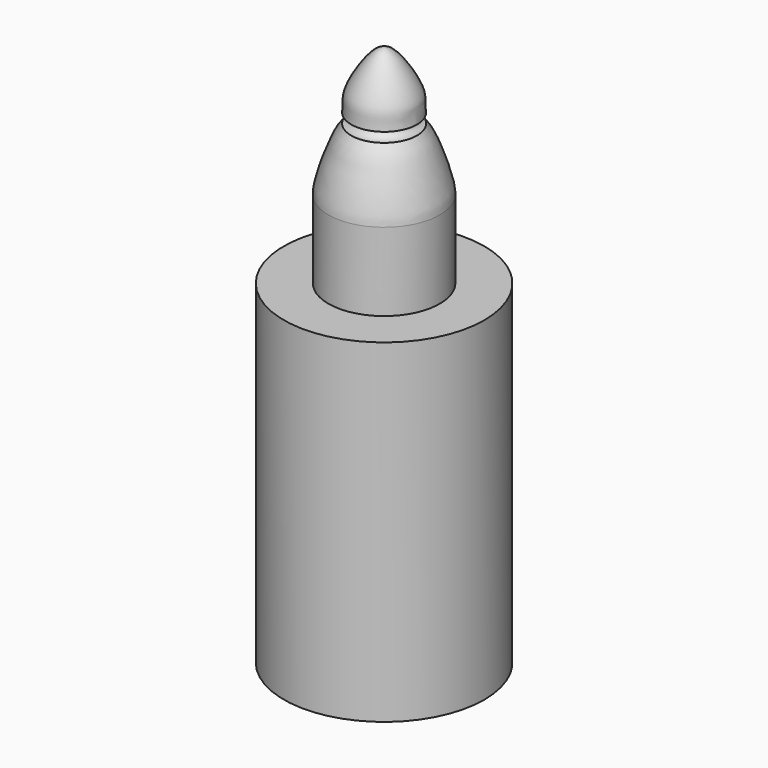
from build123d import *

# Parameters (mm, degrees)
F0_R     = 4.5
F1_DEPTH = 15


# Not quite as in the source:
# - the dataset's text gives a spline's control points without its knots; the knots are read off the source's solid


with BuildPart() as f1:
    # F0 (on Top) → F1 (new body)
    with BuildSketch(Plane.XY):
        Circle(F0_R)
    extrude(amount=F1_DEPTH)

    # F2 (on Front) → F4 (revolve)
    with BuildSketch(Plane.XZ):
        with BuildLine():
            Line((-2.5, 17.0236378187), (-2.5, 15))
            Line((-2.5, 15), (0, 15))
            Line((0, 15), (0, 24.3299212307))
            add(Edge.make_bspline(
                [(-1.4731750125, 21.747386083), (-1.435555902, 22.2030915852), (-1.5699992439, 22.5508063144), (-0.470992112, 24.2475331198), (-0.1305283548, 24.2939986482), (0, 24.3299212307)],
                knots=[0, 0, 0, 0, 0.3248303088, 0.7742925173, 1, 1, 1, 1], degree=3))
            Line((-1.4731750125, 21.747386083), (-1.0478706099, 21.8402482569))
            ThreePointArc((-1.0478706099, 21.8402482569), (-1.13410837, 21.4743640506), (-1.4731750125, 21.3120618151))
            add(Edge.make_bspline(
                [(-1.4731750125, 21.3120618151), (-1.6639285941, 21.09941035), (-2.015160403, 20.4471243002), (-2.4985771216, 18.8748984466), (-2.4986425287, 18.5918404637), (-2.5, 18.5097083037)],
                knots=[0, 0, 0, 0, 0.3554623403, 0.8005748232, 1, 1, 1, 1], degree=3))
            Line((-2.5, 18.5097083037), (-2.5, 17.0236378187))
        make_face()
    revolve(axis=Axis((0, 0, 19.6649606153), (0, 0, -1)))

    # F3 (on Right) → F5 (revolve, cut)
    with BuildSketch(Plane.YZ):
        with BuildLine():
            Line((-2.6520751002, 3.5121871486), (-2.6520751002, 0))
            Line((-2.6520751002, 0), (-0.0020955838, 0))
            Line((-0.0020955838, 0), (-0.0020955838, 9.3299212307))
            Line((-0.0020955838, 9.3299212307), (-0.0020955838, 9.4825128466))
            add(Edge.make_bspline(
                [(-0.0418971612, 9.4745443078), (-0.0286299688, 9.4772004874), (-0.0153627763, 9.479856667), (-0.0020955838, 9.4825128466)],
                knots=[0, 0, 0, 0, 0.0405914175, 0.0405914175, 0.0405914175, 0.0405914175], degree=3))
            add(Edge.make_bspline(
                [(-1.6247620893, 6.7597268096), (-1.6107579242, 6.9293686489), (-1.6097454797, 7.1757108124), (-1.6014936754, 7.4336104918), (-1.5377256315, 7.6737625858), (-1.4241040834, 7.9501711638), (-1.2053167679, 8.3534142494), (-0.8804919745, 8.8395045704), (-0.610871653, 9.1644327873), (-0.4122233725, 9.3319830663), (-0.271880498, 9.407983915), (-0.14522978, 9.4486638159), (-0.0750391264, 9.4654233396), (-0.0418971612, 9.4745443078)],
                knots=[1e-10, 1e-10, 1e-10, 1e-10, 0.1250000001, 0.2500000001, 0.3125000001, 0.3750000001, 0.5000000001, 0.625, 0.75, 0.8125, 0.875, 0.9375, 0.9999999868, 0.9999999868, 0.9999999868, 0.9999999868], degree=3))
            Line((-1.6247620893, 6.7597268096), (-1.6247620893, 6.5499318036))
            Line((-1.6247620893, 6.5499318036), (-1.4465873744, 6.6681100428))
            ThreePointArc((-1.4465873744, 6.6681100428), (-1.4480273893, 6.5854670799), (-1.4779550172, 6.5084198862))
            Line((-1.4779550172, 6.5084198862), (-1.5869297684, 6.412222832))
            add(Edge.make_bspline(
                [(-1.5869297684, 6.412222832), (-1.6603632806, 6.3303593941), (-1.7960029257, 6.1476843808), (-1.9773555127, 5.8113183689), (-2.1514419755, 5.3994309481), (-2.3273731924, 4.9091910143), (-2.4831356042, 4.4142141117), (-2.5795599889, 4.0543493292), (-2.6264757112, 3.8293515742), (-2.6506112062, 3.6534928188), (-2.6512422307, 3.5625789082), (-2.6520751002, 3.5121871486)],
                knots=[3.9e-09, 3.9e-09, 3.9e-09, 3.9e-09, 0.125, 0.2499999999, 0.3749999999, 0.4999999999, 0.6249999999, 0.7499999998, 0.8124999998, 0.8749999998, 0.9999999998, 0.9999999998, 0.9999999998, 0.9999999998], degree=3))
        make_face()
    revolve(axis=Axis((0, -0.0020955838, 4.6649606153), (0, 0, -1)), mode=Mode.SUBTRACT)


solid = f1.part
